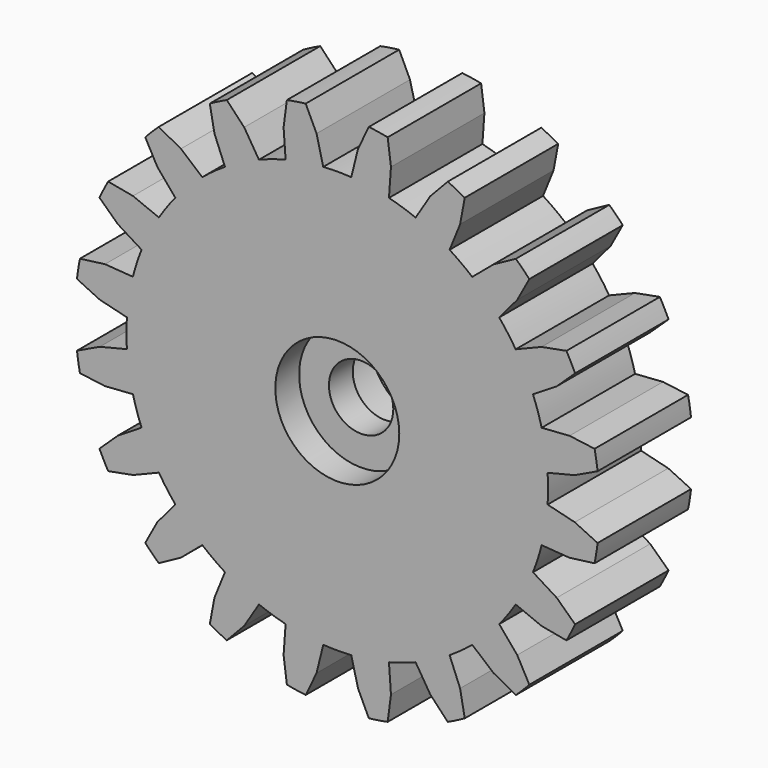
from build123d import *

# Parameters (mm, degrees)
F0_W     = 3.175
F0_H     = 3.175
F3_DEPTH = 15.875
F4_DEPTH = 0.254


# Not quite as in the source:
# - a feature names something its author has since deleted; it is built from what else it names


with BuildPart() as f1:
    # F0 (on Top) → F1 (revolve)
    with BuildSketch(Plane.XY):
        Polygon((50.8, 6.35), (6.604, 6.35), (6.604, 0), (6.604, -3.175), (6.604, -6.35), (50.8, -6.35), align=None)
        with Locations((5.0165, -1.5875)):
            Rectangle(F0_W, F0_H)
    revolve(axis=Axis((0, 0, 0), (0, -1, 0)))

    # F2 (on face) → F3 (cut)
    with BuildSketch(Plane(origin=(0, 6.35, 0), x_dir=(-1, 0, 0), z_dir=(0, 1, 0))):
        with BuildLine():
            ThreePointArc((50.7688754652, -1.778), (50.7922182703, -0.8891362011), (50.8, 0))
            ThreePointArc((50.8, 0), (50.7922182703, 0.8891362011), (50.7688754652, 1.778))
            ThreePointArc((50.7688754652, 1.778), (50.7595112733, 2.0278104688), (50.7489178855, 2.2775718321))
            ThreePointArc((50.7489178855, 2.2775718321), (50.6471260885, 3.9380983959), (50.4910157661, 5.5944013895))
            ThreePointArc((50.4910157661, 5.5944013895), (50.4573580358, 5.8902478768), (50.4219668409, 6.1858920045))
            ThreePointArc((50.4219668409, 6.1858920045), (50.1745677022, 7.946870824), (49.8656858833, 9.6981117437))
            ThreePointArc((49.8656858833, 9.6981117437), (49.3963919562, 11.8590244839), (48.8335020521, 13.9974668181))
            ThreePointArc((48.8335020521, 13.9974668181), (48.3136710278, 15.6980633142), (47.7346376201, 17.37942379))
            ThreePointArc((47.7346376201, 17.37942379), (46.9330802516, 19.4403183641), (46.0425943737, 21.4643775436))
            ThreePointArc((46.0425943737, 21.4643775436), (45.2631314288, 23.0627173868), (44.4282041567, 24.6327967437))
            ThreePointArc((44.4282041567, 24.6327967437), (43.3141203492, 26.5429270876), (42.1179652152, 28.4027640579))
            ThreePointArc((42.1179652152, 28.4027640579), (41.0980633142, 29.8594908165), (40.0278008581, 31.2796284899))
            ThreePointArc((40.0278008581, 31.2796284899), (38.6286230525, 32.9919608552), (37.1562519716, 34.6417802577))
            ThreePointArc((37.1562519716, 34.6417802577), (35.9210244843, 35.9210244843), (34.6417802577, 37.1562519716))
            ThreePointArc((34.6417802577, 37.1562519716), (32.9919608552, 38.6286230525), (31.2796284899, 40.0278008581))
            ThreePointArc((31.2796284899, 40.0278008581), (29.8594908165, 41.0980633142), (28.4027640579, 42.1179652152))
            ThreePointArc((28.4027640579, 42.1179652152), (26.5429270876, 43.3141203492), (24.6327967437, 44.4282041567))
            ThreePointArc((24.6327967437, 44.4282041567), (23.0627173868, 45.2631314288), (21.4643775436, 46.0425943737))
            ThreePointArc((21.4643775436, 46.0425943737), (19.4403183641, 46.9330802516), (17.37942379, 47.7346376201))
            ThreePointArc((17.37942379, 47.7346376201), (15.6980633142, 48.3136710278), (13.9974668181, 48.8335020521))
            ThreePointArc((13.9974668181, 48.8335020521), (11.8590244839, 49.3963919562), (9.6981117437, 49.8656858833))
            ThreePointArc((9.6981117437, 49.8656858833), (7.946870824, 50.1745677022), (6.1858920045, 50.4219668409))
            ThreePointArc((6.1858920045, 50.4219668409), (3.985722063, 50.6434005536), (1.778, 50.7688754652))
            ThreePointArc((1.778, 50.7688754652), (0, 50.8), (-1.778, 50.7688754652))
            ThreePointArc((-1.778, 50.7688754652), (-3.985722063, 50.6434005536), (-6.1858920045, 50.4219668409))
            ThreePointArc((-6.1858920045, 50.4219668409), (-7.946870824, 50.1745677022), (-9.6981117437, 49.8656858833))
            ThreePointArc((-9.6981117437, 49.8656858833), (-11.8590244839, 49.3963919562), (-13.9974668181, 48.8335020521))
            ThreePointArc((-13.9974668181, 48.8335020521), (-15.6980633142, 48.3136710278), (-17.37942379, 47.7346376201))
            ThreePointArc((-17.37942379, 47.7346376201), (-19.4403183641, 46.9330802516), (-21.4643775436, 46.0425943737))
            ThreePointArc((-21.4643775436, 46.0425943737), (-23.0627173868, 45.2631314288), (-24.6327967437, 44.4282041567))
            ThreePointArc((-24.6327967437, 44.4282041567), (-26.5429270876, 43.3141203492), (-28.4027640579, 42.1179652152))
            ThreePointArc((-28.4027640579, 42.1179652152), (-29.8594908165, 41.0980633142), (-31.2796284899, 40.0278008581))
            ThreePointArc((-31.2796284899, 40.0278008581), (-32.9919608552, 38.6286230525), (-34.6417802577, 37.1562519716))
            ThreePointArc((-34.6417802577, 37.1562519716), (-35.9210244843, 35.9210244843), (-37.1562519716, 34.6417802577))
            ThreePointArc((-37.1562519716, 34.6417802577), (-38.6286230525, 32.9919608552), (-40.0278008581, 31.2796284899))
            ThreePointArc((-40.0278008581, 31.2796284899), (-41.0980633142, 29.8594908165), (-42.1179652152, 28.4027640579))
            ThreePointArc((-42.1179652152, 28.4027640579), (-43.3141203492, 26.5429270876), (-44.4282041567, 24.6327967437))
            ThreePointArc((-44.4282041567, 24.6327967437), (-45.2631314288, 23.0627173868), (-46.0425943737, 21.4643775436))
            ThreePointArc((-46.0425943737, 21.4643775436), (-46.9330802516, 19.4403183641), (-47.7346376201, 17.37942379))
            ThreePointArc((-47.7346376201, 17.37942379), (-48.3136710278, 15.6980633142), (-48.8335020521, 13.9974668181))
            ThreePointArc((-48.8335020521, 13.9974668181), (-49.3963919562, 11.8590244839), (-49.8656858833, 9.6981117437))
            ThreePointArc((-49.8656858833, 9.6981117437), (-50.1745677022, 7.946870824), (-50.4219668409, 6.1858920045))
            ThreePointArc((-50.4219668409, 6.1858920045), (-50.6434005536, 3.985722063), (-50.7688754652, 1.778))
            ThreePointArc((-50.7688754652, 1.778), (-50.8, 0), (-50.7688754652, -1.778))
            ThreePointArc((-50.7688754652, -1.778), (-50.6434005536, -3.985722063), (-50.4219668409, -6.1858920045))
            ThreePointArc((-50.4219668409, -6.1858920045), (-50.1745677022, -7.946870824), (-49.8656858833, -9.6981117437))
            ThreePointArc((-49.8656858833, -9.6981117437), (-49.3963919562, -11.8590244839), (-48.8335020521, -13.9974668181))
            ThreePointArc((-48.8335020521, -13.9974668181), (-48.3136710278, -15.6980633142), (-47.7346376201, -17.37942379))
            ThreePointArc((-47.7346376201, -17.37942379), (-46.9330802516, -19.4403183641), (-46.0425943737, -21.4643775436))
            ThreePointArc((-46.0425943737, -21.4643775436), (-45.2631314288, -23.0627173868), (-44.4282041567, -24.6327967437))
            ThreePointArc((-44.4282041567, -24.6327967437), (-43.3141203492, -26.5429270876), (-42.1179652152, -28.4027640579))
            ThreePointArc((-42.1179652152, -28.4027640579), (-41.0980633142, -29.8594908165), (-40.0278008581, -31.2796284899))
            ThreePointArc((-40.0278008581, -31.2796284899), (-38.6286230525, -32.9919608552), (-37.1562519716, -34.6417802577))
            ThreePointArc((-37.1562519716, -34.6417802577), (-35.9210244843, -35.9210244843), (-34.6417802577, -37.1562519716))
            ThreePointArc((-34.6417802577, -37.1562519716), (-32.9919608552, -38.6286230525), (-31.2796284899, -40.0278008581))
            ThreePointArc((-31.2796284899, -40.0278008581), (-29.8594908165, -41.0980633142), (-28.4027640579, -42.1179652152))
            ThreePointArc((-28.4027640579, -42.1179652152), (-26.5429270876, -43.3141203492), (-24.6327967437, -44.4282041567))
            ThreePointArc((-24.6327967437, -44.4282041567), (-23.0627173868, -45.2631314288), (-21.4643775436, -46.0425943737))
            ThreePointArc((-21.4643775436, -46.0425943737), (-19.4403183641, -46.9330802516), (-17.37942379, -47.7346376201))
            ThreePointArc((-17.37942379, -47.7346376201), (-15.6980633142, -48.3136710278), (-13.9974668181, -48.8335020521))
            ThreePointArc((-13.9974668181, -48.8335020521), (-11.8590244839, -49.3963919562), (-9.6981117437, -49.8656858833))
            ThreePointArc((-9.6981117437, -49.8656858833), (-7.946870824, -50.1745677022), (-6.1858920045, -50.4219668409))
            ThreePointArc((-6.1858920045, -50.4219668409), (-3.985722063, -50.6434005536), (-1.778, -50.7688754652))
            ThreePointArc((-1.778, -50.7688754652), (0, -50.8), (1.778, -50.7688754652))
            ThreePointArc((1.778, -50.7688754652), (3.985722063, -50.6434005536), (6.1858920045, -50.4219668409))
            ThreePointArc((6.1858920045, -50.4219668409), (7.946870824, -50.1745677022), (9.6981117437, -49.8656858833))
            ThreePointArc((9.6981117437, -49.8656858833), (11.8590244839, -49.3963919562), (13.9974668181, -48.8335020521))
            ThreePointArc((13.9974668181, -48.8335020521), (15.6980633142, -48.3136710278), (17.37942379, -47.7346376201))
            ThreePointArc((17.37942379, -47.7346376201), (19.4403183641, -46.9330802516), (21.4643775436, -46.0425943737))
            ThreePointArc((21.4643775436, -46.0425943737), (23.0627173868, -45.2631314288), (24.6327967437, -44.4282041567))
            ThreePointArc((24.6327967437, -44.4282041567), (26.5429270876, -43.3141203492), (28.4027640579, -42.1179652152))
            ThreePointArc((28.4027640579, -42.1179652152), (29.8594908165, -41.0980633142), (31.2796284899, -40.0278008581))
            ThreePointArc((31.2796284899, -40.0278008581), (32.9919608552, -38.6286230525), (34.6417802577, -37.1562519716))
            ThreePointArc((34.6417802577, -37.1562519716), (35.9210244843, -35.9210244843), (37.1562519716, -34.6417802577))
            ThreePointArc((37.1562519716, -34.6417802577), (38.6286230525, -32.9919608552), (40.0278008581, -31.2796284899))
            ThreePointArc((40.0278008581, -31.2796284899), (41.0980633142, -29.8594908165), (42.1179652152, -28.4027640579))
            ThreePointArc((42.1179652152, -28.4027640579), (43.3141203492, -26.5429270876), (44.4282041567, -24.6327967437))
            ThreePointArc((44.4282041567, -24.6327967437), (45.2631314288, -23.0627173868), (46.0425943737, -21.4643775436))
            ThreePointArc((46.0425943737, -21.4643775436), (46.9330802516, -19.4403183641), (47.7346376201, -17.37942379))
            ThreePointArc((47.7346376201, -17.37942379), (48.3136710278, -15.6980633142), (48.8335020521, -13.9974668181))
            ThreePointArc((48.8335020521, -13.9974668181), (49.3963919562, -11.8590244839), (49.8656858833, -9.6981117437))
            ThreePointArc((49.8656858833, -9.6981117437), (50.1745677022, -7.946870824), (50.4219668409, -6.1858920045))
            ThreePointArc((50.4219668409, -6.1858920045), (50.4573580358, -5.8902478768), (50.4910157661, -5.5944013895))
            ThreePointArc((50.4910157661, -5.5944013895), (50.6471260885, -3.9380983959), (50.7489178855, -2.2775718321))
            ThreePointArc((50.7489178855, -2.2775718321), (50.7595112733, -2.0278104688), (50.7688754652, -1.778))
        make_face()
        with BuildLine():
            ThreePointArc((27.7366983199, 3.364396872), (27.8891282676, 1.6852668843), (27.94, 0))
            ThreePointArc((27.94, 0), (27.8891282676, -1.6852668843), (27.7366983199, -3.364396872))
            ThreePointArc((27.7366983199, -3.364396872), (27.5960122362, -4.3707789532), (27.4188234869, -5.3713795801))
            ThreePointArc((27.4188234869, -5.3713795801), (26.5725190653, -8.6339348228), (25.3395118683, -11.7708427172))
            ThreePointArc((25.3395118683, -11.7708427172), (24.8947222858, -12.6844945627), (24.4170031729, -13.5813679744))
            ThreePointArc((24.4170031729, -13.5813679744), (22.6039348228, -16.4227199491), (20.4619174444, -19.025076465))
            ThreePointArc((20.4619174444, -19.025076465), (19.7565634664, -19.7565634664), (19.025076465, -20.4619174444))
            ThreePointArc((19.025076465, -20.4619174444), (16.4227199491, -22.6039348228), (13.5813679744, -24.4170031729))
            ThreePointArc((13.5813679744, -24.4170031729), (12.6844945627, -24.8947222858), (11.7708427172, -25.3395118683))
            ThreePointArc((11.7708427172, -25.3395118683), (8.6339348228, -26.5725190653), (5.3713795801, -27.4188234869))
            ThreePointArc((5.3713795801, -27.4188234869), (4.3707789532, -27.5960122362), (3.364396872, -27.7366983199))
            ThreePointArc((3.364396872, -27.7366983199), (1.6852668843, -27.8891282676), (0, -27.94))
            ThreePointArc((0, -27.94), (-1.6852668843, -27.8891282676), (-3.364396872, -27.7366983199))
            ThreePointArc((-3.364396872, -27.7366983199), (-4.3707789532, -27.5960122362), (-5.3713795801, -27.4188234869))
            ThreePointArc((-5.3713795801, -27.4188234869), (-8.6339348228, -26.5725190653), (-11.7708427172, -25.3395118683))
            ThreePointArc((-11.7708427172, -25.3395118683), (-12.6844945627, -24.8947222858), (-13.5813679744, -24.4170031729))
            ThreePointArc((-13.5813679744, -24.4170031729), (-16.4227199491, -22.6039348228), (-19.025076465, -20.4619174444))
            ThreePointArc((-19.025076465, -20.4619174444), (-19.7565634664, -19.7565634664), (-20.4619174444, -19.025076465))
            ThreePointArc((-20.4619174444, -19.025076465), (-22.6039348228, -16.4227199491), (-24.4170031729, -13.5813679744))
            ThreePointArc((-24.4170031729, -13.5813679744), (-24.8947222858, -12.6844945627), (-25.3395118683, -11.7708427172))
            ThreePointArc((-25.3395118683, -11.7708427172), (-26.5725190653, -8.6339348228), (-27.4188234869, -5.3713795801))
            ThreePointArc((-27.4188234869, -5.3713795801), (-27.5960122362, -4.3707789532), (-27.7366983199, -3.364396872))
            ThreePointArc((-27.7366983199, -3.364396872), (-27.94, 0), (-27.7366983199, 3.364396872))
            ThreePointArc((-27.7366983199, 3.364396872), (-27.5960122362, 4.3707789532), (-27.4188234869, 5.3713795801))
            ThreePointArc((-27.4188234869, 5.3713795801), (-26.5725190653, 8.6339348228), (-25.3395118683, 11.7708427172))
            ThreePointArc((-25.3395118683, 11.7708427172), (-24.8947222858, 12.6844945627), (-24.4170031729, 13.5813679744))
            ThreePointArc((-24.4170031729, 13.5813679744), (-22.6039348228, 16.4227199491), (-20.4619174444, 19.025076465))
            ThreePointArc((-20.4619174444, 19.025076465), (-19.7565634664, 19.7565634664), (-19.025076465, 20.4619174444))
            ThreePointArc((-19.025076465, 20.4619174444), (-16.4227199491, 22.6039348228), (-13.5813679744, 24.4170031729))
            ThreePointArc((-13.5813679744, 24.4170031729), (-12.6844945627, 24.8947222858), (-11.7708427172, 25.3395118683))
            ThreePointArc((-11.7708427172, 25.3395118683), (-8.6339348228, 26.5725190653), (-5.3713795801, 27.4188234869))
            ThreePointArc((-5.3713795801, 27.4188234869), (-4.3707789532, 27.5960122362), (-3.364396872, 27.7366983199))
            ThreePointArc((-3.364396872, 27.7366983199), (0, 27.94), (3.364396872, 27.7366983199))
            ThreePointArc((3.364396872, 27.7366983199), (4.3707789532, 27.5960122362), (5.3713795801, 27.4188234869))
            ThreePointArc((5.3713795801, 27.4188234869), (8.6339348228, 26.5725190653), (11.7708427172, 25.3395118683))
            ThreePointArc((11.7708427172, 25.3395118683), (12.6844945627, 24.8947222858), (13.5813679744, 24.4170031729))
            ThreePointArc((13.5813679744, 24.4170031729), (16.4227199491, 22.6039348228), (19.025076465, 20.4619174444))
            ThreePointArc((19.025076465, 20.4619174444), (19.7565634664, 19.7565634664), (20.4619174444, 19.025076465))
            ThreePointArc((20.4619174444, 19.025076465), (22.6039348228, 16.4227199491), (24.4170031729, 13.5813679744))
            ThreePointArc((24.4170031729, 13.5813679744), (24.8947222858, 12.6844945627), (25.3395118683, 11.7708427172))
            ThreePointArc((25.3395118683, 11.7708427172), (26.5725190653, 8.6339348228), (27.4188234869, 5.3713795801))
            ThreePointArc((27.4188234869, 5.3713795801), (27.5960122362, 4.3707789532), (27.7366983199, 3.364396872))
        make_face(mode=Mode.SUBTRACT)
        with BuildLine():
            Line((-19.1736908076, 16.6592190937), (-20.4619174444, 19.025076465))
            ThreePointArc((-20.4619174444, 19.025076465), (-22.6039348228, 16.4227199491), (-24.4170031729, 13.5813679744))
            Line((-24.4170031729, 13.5813679744), (-21.7688551799, 13.0872817711))
            Line((-21.7688551799, 13.0872817711), (-19.0085201837, 11.9658917057))
            ThreePointArc((-19.0085201837, 11.9658917057), (-18.1715086944, 13.2023738645), (-17.2541950547, 14.380513096))
            Line((-17.2541950547, 14.380513096), (-19.1736908076, 16.6592190937))
        make_face()
        with BuildLine():
            Line((-13.0872817711, 21.7688551799), (-13.5813679744, 24.4170031729))
            ThreePointArc((-13.5813679744, 24.4170031729), (-16.4227199491, 22.6039348228), (-19.025076465, 20.4619174444))
            Line((-19.025076465, 20.4619174444), (-16.6592190937, 19.1736908076))
            Line((-16.6592190937, 19.1736908076), (-14.380513096, 17.2541950547))
            ThreePointArc((-14.380513096, 17.2541950547), (-13.2023738645, 18.1715086944), (-11.9658917057, 19.0085201837))
            Line((-11.9658917057, 19.0085201837), (-13.0872817711, 21.7688551799))
        make_face()
        with BuildLine():
            Line((-5.7197984103, 24.7476040486), (-5.3713795801, 27.4188234869))
            ThreePointArc((-5.3713795801, 27.4188234869), (-8.6339348228, 26.5725190653), (-11.7708427172, 25.3395118683))
            Line((-11.7708427172, 25.3395118683), (-9.918862571, 23.383245397))
            Line((-9.918862571, 23.383245397), (-8.3448411914, 20.8535375747))
            ThreePointArc((-8.3448411914, 20.8535375747), (-6.9408986944, 21.3618896449), (-5.5062835053, 21.7758408758))
            Line((-5.5062835053, 21.7758408758), (-5.7197984103, 24.7476040486))
        make_face()
        with BuildLine():
            Line((2.2075786711, 25.3038850063), (3.364396872, 27.7366983199))
            ThreePointArc((3.364396872, 27.7366983199), (0, 27.94), (-3.364396872, 27.7366983199))
            Line((-3.364396872, 27.7366983199), (-2.2075786711, 25.3038850063))
            Line((-2.2075786711, 25.3038850063), (-1.4923180891, 22.4115905417))
            ThreePointArc((-1.4923180891, 22.4115905417), (0, 22.46122), (1.4923180891, 22.4115905417))
            Line((1.4923180891, 22.4115905417), (2.2075786711, 25.3038850063))
        make_face()
        with BuildLine():
            Line((9.918862571, 23.383245397), (11.7708427172, 25.3395118683))
            ThreePointArc((11.7708427172, 25.3395118683), (8.6339348228, 26.5725190653), (5.3713795801, 27.4188234869))
            Line((5.3713795801, 27.4188234869), (5.7197984103, 24.7476040486))
            Line((5.7197984103, 24.7476040486), (5.5062835053, 21.7758408758))
            ThreePointArc((5.5062835053, 21.7758408758), (6.9408986944, 21.3618896449), (8.3448411914, 20.8535375747))
            Line((8.3448411914, 20.8535375747), (9.918862571, 23.383245397))
        make_face()
        with BuildLine():
            Line((16.6592190937, 19.1736908076), (19.025076465, 20.4619174444))
            ThreePointArc((19.025076465, 20.4619174444), (16.4227199491, 22.6039348228), (13.5813679744, 24.4170031729))
            Line((13.5813679744, 24.4170031729), (13.0872817711, 21.7688551799))
            Line((13.0872817711, 21.7688551799), (11.9658917057, 19.0085201837))
            ThreePointArc((11.9658917057, 19.0085201837), (13.2023738645, 18.1715086944), (14.380513096, 17.2541950547))
            Line((14.380513096, 17.2541950547), (16.6592190937, 19.1736908076))
        make_face()
        with BuildLine():
            Line((21.7688551799, 13.0872817711), (24.4170031729, 13.5813679744))
            ThreePointArc((24.4170031729, 13.5813679744), (22.6039348228, 16.4227199491), (20.4619174444, 19.025076465))
            Line((20.4619174444, 19.025076465), (19.1736908076, 16.6592190937))
            Line((19.1736908076, 16.6592190937), (17.2541950547, 14.380513096))
            ThreePointArc((17.2541950547, 14.380513096), (18.1715086944, 13.2023738645), (19.0085201837, 11.9658917057))
            Line((19.0085201837, 11.9658917057), (21.7688551799, 13.0872817711))
        make_face()
        with BuildLine():
            Line((24.7476040486, 5.7197984103), (27.4188234869, 5.3713795801))
            ThreePointArc((27.4188234869, 5.3713795801), (26.5725190653, 8.6339348228), (25.3395118683, 11.7708427172))
            Line((25.3395118683, 11.7708427172), (23.383245397, 9.918862571))
            Line((23.383245397, 9.918862571), (20.8535375747, 8.3448411914))
            ThreePointArc((20.8535375747, 8.3448411914), (21.3618896449, 6.9408986944), (21.7758408758, 5.5062835053))
            Line((21.7758408758, 5.5062835053), (24.7476040486, 5.7197984103))
        make_face()
        with BuildLine():
            ThreePointArc((27.7366983199, -3.364396872), (27.8891282676, -1.6852668843), (27.94, 0))
            ThreePointArc((27.94, 0), (27.8891282676, 1.6852668843), (27.7366983199, 3.364396872))
            Line((27.7366983199, 3.364396872), (25.3038850063, 2.2075786711))
            Line((25.3038850063, 2.2075786711), (22.4115905417, 1.4923180891))
            ThreePointArc((22.4115905417, 1.4923180891), (22.4488092067, 0.7465715576), (22.46122, 0))
            ThreePointArc((22.46122, 0), (22.4488092067, -0.7465715576), (22.4115905417, -1.4923180891))
            Line((22.4115905417, -1.4923180891), (25.3038850063, -2.2075786711))
            Line((25.3038850063, -2.2075786711), (27.7366983199, -3.364396872))
        make_face()
        with BuildLine():
            ThreePointArc((25.3395118683, -11.7708427172), (26.5725190653, -8.6339348228), (27.4188234869, -5.3713795801))
            Line((27.4188234869, -5.3713795801), (24.7476040486, -5.7197984103))
            Line((24.7476040486, -5.7197984103), (21.7758408758, -5.5062835053))
            ThreePointArc((21.7758408758, -5.5062835053), (21.3618896449, -6.9408986944), (20.8535375747, -8.3448411914))
            Line((20.8535375747, -8.3448411914), (23.383245397, -9.918862571))
            Line((23.383245397, -9.918862571), (25.3395118683, -11.7708427172))
        make_face()
        with BuildLine():
            ThreePointArc((20.4619174444, -19.025076465), (22.6039348228, -16.4227199491), (24.4170031729, -13.5813679744))
            Line((24.4170031729, -13.5813679744), (21.7688551799, -13.0872817711))
            Line((21.7688551799, -13.0872817711), (19.0085201837, -11.9658917057))
            ThreePointArc((19.0085201837, -11.9658917057), (18.1715086944, -13.2023738645), (17.2541950547, -14.380513096))
            Line((17.2541950547, -14.380513096), (19.1736908076, -16.6592190937))
            Line((19.1736908076, -16.6592190937), (20.4619174444, -19.025076465))
        make_face()
        with BuildLine():
            ThreePointArc((13.5813679744, -24.4170031729), (16.4227199491, -22.6039348228), (19.025076465, -20.4619174444))
            Line((19.025076465, -20.4619174444), (16.6592190937, -19.1736908076))
            Line((16.6592190937, -19.1736908076), (14.380513096, -17.2541950547))
            ThreePointArc((14.380513096, -17.2541950547), (13.2023738645, -18.1715086944), (11.9658917057, -19.0085201837))
            Line((11.9658917057, -19.0085201837), (13.0872817711, -21.7688551799))
            Line((13.0872817711, -21.7688551799), (13.5813679744, -24.4170031729))
        make_face()
        with BuildLine():
            ThreePointArc((5.3713795801, -27.4188234869), (8.6339348228, -26.5725190653), (11.7708427172, -25.3395118683))
            Line((11.7708427172, -25.3395118683), (9.918862571, -23.383245397))
            Line((9.918862571, -23.383245397), (8.3448411914, -20.8535375747))
            ThreePointArc((8.3448411914, -20.8535375747), (6.9408986944, -21.3618896449), (5.5062835053, -21.7758408758))
            Line((5.5062835053, -21.7758408758), (5.7197984103, -24.7476040486))
            Line((5.7197984103, -24.7476040486), (5.3713795801, -27.4188234869))
        make_face()
        with BuildLine():
            ThreePointArc((-11.7708427172, -25.3395118683), (-8.6339348228, -26.5725190653), (-5.3713795801, -27.4188234869))
            Line((-5.3713795801, -27.4188234869), (-5.7197984103, -24.7476040486))
            Line((-5.7197984103, -24.7476040486), (-5.5062835053, -21.7758408758))
            ThreePointArc((-5.5062835053, -21.7758408758), (-6.9408986944, -21.3618896449), (-8.3448411914, -20.8535375747))
            Line((-8.3448411914, -20.8535375747), (-9.918862571, -23.383245397))
            Line((-9.918862571, -23.383245397), (-11.7708427172, -25.3395118683))
        make_face()
        with BuildLine():
            ThreePointArc((-19.025076465, -20.4619174444), (-16.4227199491, -22.6039348228), (-13.5813679744, -24.4170031729))
            Line((-13.5813679744, -24.4170031729), (-13.0872817711, -21.7688551799))
            Line((-13.0872817711, -21.7688551799), (-11.9658917057, -19.0085201837))
            ThreePointArc((-11.9658917057, -19.0085201837), (-13.2023738645, -18.1715086944), (-14.380513096, -17.2541950547))
            Line((-14.380513096, -17.2541950547), (-16.6592190937, -19.1736908076))
            Line((-16.6592190937, -19.1736908076), (-19.025076465, -20.4619174444))
        make_face()
        with BuildLine():
            ThreePointArc((-24.4170031729, -13.5813679744), (-22.6039348228, -16.4227199491), (-20.4619174444, -19.025076465))
            Line((-20.4619174444, -19.025076465), (-19.1736908076, -16.6592190937))
            Line((-19.1736908076, -16.6592190937), (-17.2541950547, -14.380513096))
            ThreePointArc((-17.2541950547, -14.380513096), (-18.1715086944, -13.2023738645), (-19.0085201837, -11.9658917057))
            Line((-19.0085201837, -11.9658917057), (-21.7688551799, -13.0872817711))
            Line((-21.7688551799, -13.0872817711), (-24.4170031729, -13.5813679744))
        make_face()
        with BuildLine():
            ThreePointArc((-27.4188234869, -5.3713795801), (-26.5725190653, -8.6339348228), (-25.3395118683, -11.7708427172))
            Line((-25.3395118683, -11.7708427172), (-23.383245397, -9.918862571))
            Line((-23.383245397, -9.918862571), (-20.8535375747, -8.3448411914))
            ThreePointArc((-20.8535375747, -8.3448411914), (-21.3618896449, -6.9408986944), (-21.7758408758, -5.5062835053))
            Line((-21.7758408758, -5.5062835053), (-24.7476040486, -5.7197984103))
            Line((-24.7476040486, -5.7197984103), (-27.4188234869, -5.3713795801))
        make_face()
        with BuildLine():
            Line((-25.3038850063, 2.2075786711), (-27.7366983199, 3.364396872))
            ThreePointArc((-27.7366983199, 3.364396872), (-27.94, 0), (-27.7366983199, -3.364396872))
            Line((-27.7366983199, -3.364396872), (-25.3038850063, -2.2075786711))
            Line((-25.3038850063, -2.2075786711), (-22.4115905417, -1.4923180891))
            ThreePointArc((-22.4115905417, -1.4923180891), (-22.46122, 0), (-22.4115905417, 1.4923180891))
            Line((-22.4115905417, 1.4923180891), (-25.3038850063, 2.2075786711))
        make_face()
        with BuildLine():
            Line((-23.383245397, 9.918862571), (-25.3395118683, 11.7708427172))
            ThreePointArc((-25.3395118683, 11.7708427172), (-26.5725190653, 8.6339348228), (-27.4188234869, 5.3713795801))
            Line((-27.4188234869, 5.3713795801), (-24.7476040486, 5.7197984103))
            Line((-24.7476040486, 5.7197984103), (-21.7758408758, 5.5062835053))
            ThreePointArc((-21.7758408758, 5.5062835053), (-21.3618896449, 6.9408986944), (-20.8535375747, 8.3448411914))
            Line((-20.8535375747, 8.3448411914), (-23.383245397, 9.918862571))
        make_face()
        with BuildLine():
            ThreePointArc((-3.364396872, -27.7366983199), (-1.6852668843, -27.8891282676), (0, -27.94))
            Line((0, -27.94), (0, -22.46122))
            ThreePointArc((0, -22.46122), (-0.7465715576, -22.4488092067), (-1.4923180891, -22.4115905417))
            Line((-1.4923180891, -22.4115905417), (-2.2075786711, -25.3038850063))
            Line((-2.2075786711, -25.3038850063), (-3.364396872, -27.7366983199))
        make_face()
        with BuildLine():
            ThreePointArc((0, -27.94), (1.6852668843, -27.8891282676), (3.364396872, -27.7366983199))
            Line((3.364396872, -27.7366983199), (2.2075786711, -25.3038850063))
            Line((2.2075786711, -25.3038850063), (1.4923180891, -22.4115905417))
            ThreePointArc((1.4923180891, -22.4115905417), (0.7465715576, -22.4488092067), (0, -22.46122))
            Line((0, -22.46122), (0, -27.94))
        make_face()
    extrude(amount=-F3_DEPTH, mode=Mode.SUBTRACT)

    # F4 (cut): a face of the model
    f4_faces = [f1.faces().sort_by_distance(p)[0] for p in [
        (23.822037879, 6.35, 11.4145640609),
    ]]
    extrude(f4_faces, amount=-F4_DEPTH, mode=Mode.SUBTRACT)


solid = f1.part
